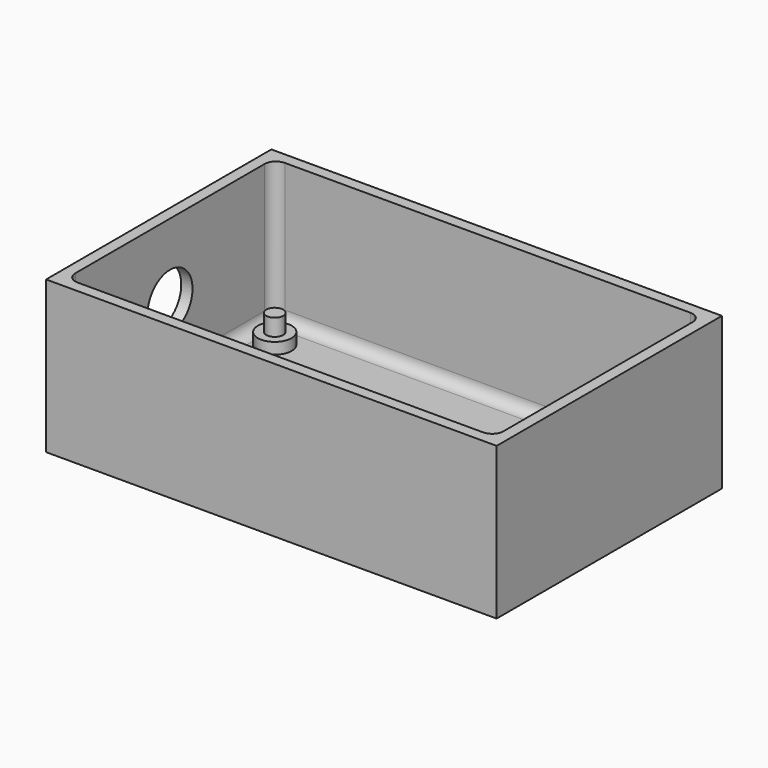
from build123d import *

# Parameters (mm, degrees)
F0_W     = 80
F0_H     = 50
F1_DEPTH = 27
F2_W     = 76
F2_H     = 46
F3_DEPTH = 25
F4_R     = 3
F5_DEPTH = 2
F6_R     = 1.5
F7_DEPTH = 3
F8_R     = 5
F9_DEPTH = 25
F10_R    = 1.99999


# Not quite as in the source:
# - a fillet or chamfer is up to 0.001 mm smaller than in the source, because OpenCascade refuses the exact size


with BuildPart() as f1:
    # F0 (on Top) → F1 (new body)
    with BuildSketch(Plane.XY):
        Rectangle(F0_W, F0_H)
    extrude(amount=F1_DEPTH)

    # F2 (on face) → F3 (cut)
    with BuildSketch(Plane.XY.offset(27)):
        Rectangle(F2_W, F2_H)
    extrude(amount=-F3_DEPTH, mode=Mode.SUBTRACT)

    # F4 (on face) → F5 (join)
    with BuildSketch(Plane.XY.offset(2)):
        with Locations((-33, 17)):
            Circle(F4_R)
        with Locations((27, 17)):
            Circle(F4_R)
        with Locations((27, -17)):
            Circle(F4_R)
        with Locations((-33, -17)):
            Circle(F4_R)
    extrude(amount=F5_DEPTH)

    # F6 (on face) → F7 (join)
    with BuildSketch(Plane.XY.offset(4)):
        with Locations((-33, 17)):
            Circle(F6_R)
        with Locations((27, 17)):
            Circle(F6_R)
        with Locations((27, -17)):
            Circle(F6_R)
        with Locations((-33, -17)):
            Circle(F6_R)
    extrude(amount=F7_DEPTH)

    # F8 (on face) → F9 (cut)
    with BuildSketch(Plane(origin=(-40, 0, 0), x_dir=(0, -1, 0), z_dir=(-1, 0, 0))):
        with Locations((0, 14)):
            Circle(F8_R)
    extrude(amount=-F9_DEPTH, mode=Mode.SUBTRACT)

    # F10 (radius 2 in the source; OpenCascade refuses exactly that, so slightly less here)
    f10_edges = [f1.edges().sort_by_distance(p)[0] for p in [
        (-38, 23, 14.5),
        (38, 23, 14.5),
        (38, -23, 14.5),
        (-38, -23, 14.5),
        (0, 23, 2),
        (38, 0, 2),
        (0, -23, 2),
        (-38, 0, 2),
    ]]
    fillet(f10_edges, radius=F10_R)


solid = f1.part
